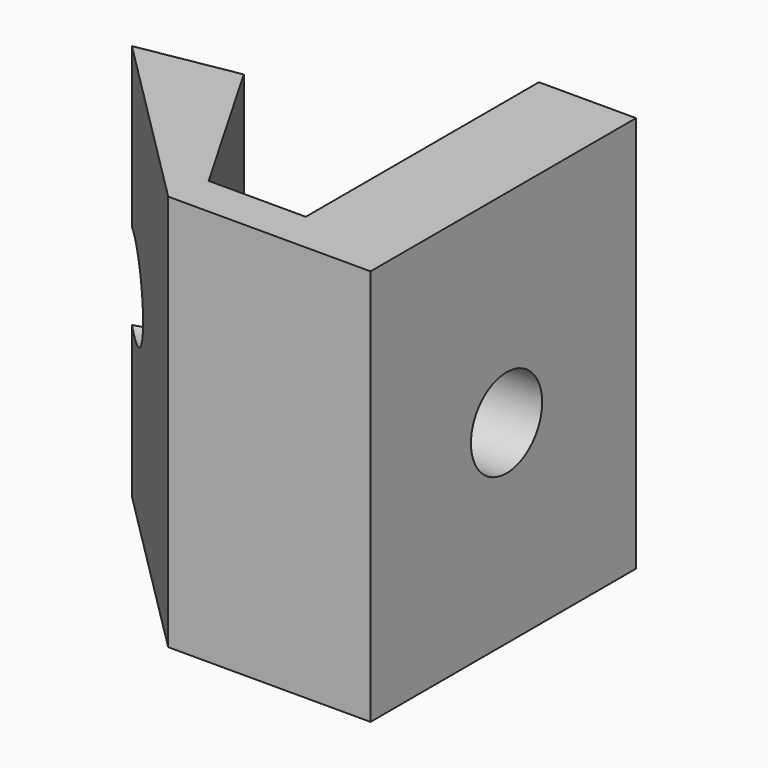
from build123d import *

# Parameters (mm, degrees)
F1_DEPTH = 9.8
F3_D     = 2.2
F3_DEPTH = 34.7787770473


with BuildPart() as f1:
    # F0 (on Top) → F1 (new body)
    with BuildSketch(Plane.XY):
        Polygon((-34.7777770473, 4.3244506916), (-30.3039783165, -0.1493480393), (-25.3039783165, -0.1493480393), (-25.3039783165, 8.0506519607), (-27.7039783165, 8.0506519607), (-27.7039783165, 0.8506519607), (-30.1039783165, 0.8506519607), (-32.3539783165, 4.7477662778), align=None)
    extrude(amount=F1_DEPTH)

    # F3 (through all, one way)
    with BuildSketch(Plane.YZ):
        with Locations((4.0506519607, 4.8)):
            Circle(F3_D / 2)
    extrude(amount=-F3_DEPTH, mode=Mode.SUBTRACT)


solid = f1.part
